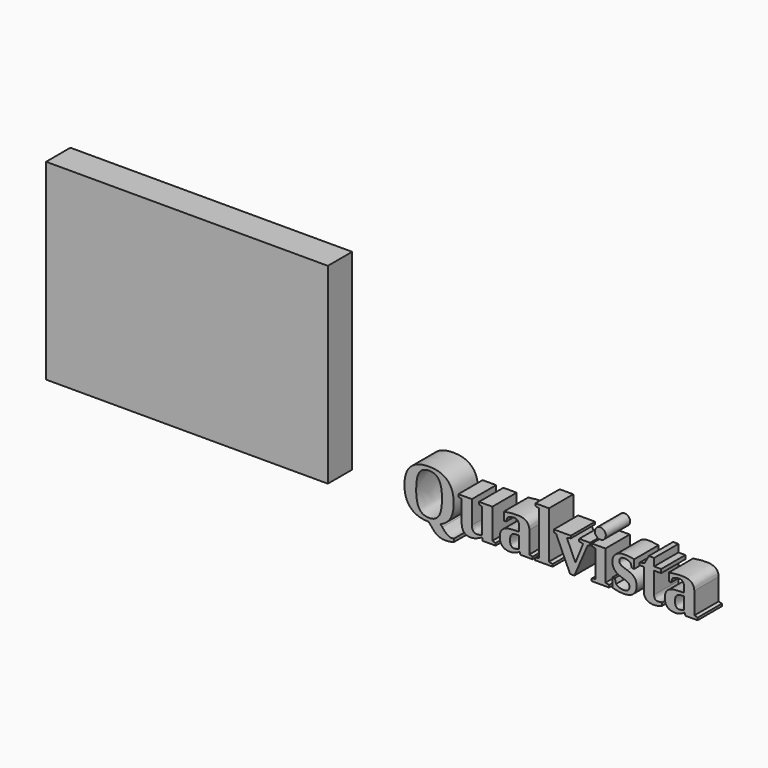
from build123d import *

# Parameters (mm, degrees)
F0_W         = 46.3839136064
F0_H         = 31.5730087459
F0_TEXT_SIZE = 11.9230076153
F1_DEPTH     = 5


# Not quite as in the source:
# - Text() gives the source's letters only with a copy of the font that has no kerning and outlines rounded to 1/6400 em; it was checked with that copy


with BuildPart() as f1:
    # F0 (on Front) → F1 (new body)
    with BuildSketch(Plane.XZ):
        with Locations((-23.1919568032, 15.786504373)):
            Rectangle(F0_W, F0_H)
        with Locations((12.0254904032, 0)):
            Text('Qualvista', F0_TEXT_SIZE, font='Tinos', font_style=FontStyle.BOLD, text_align=(TextAlign.LEFT, TextAlign.BOTTOM))
    extrude(amount=F1_DEPTH)


solid = f1.part
